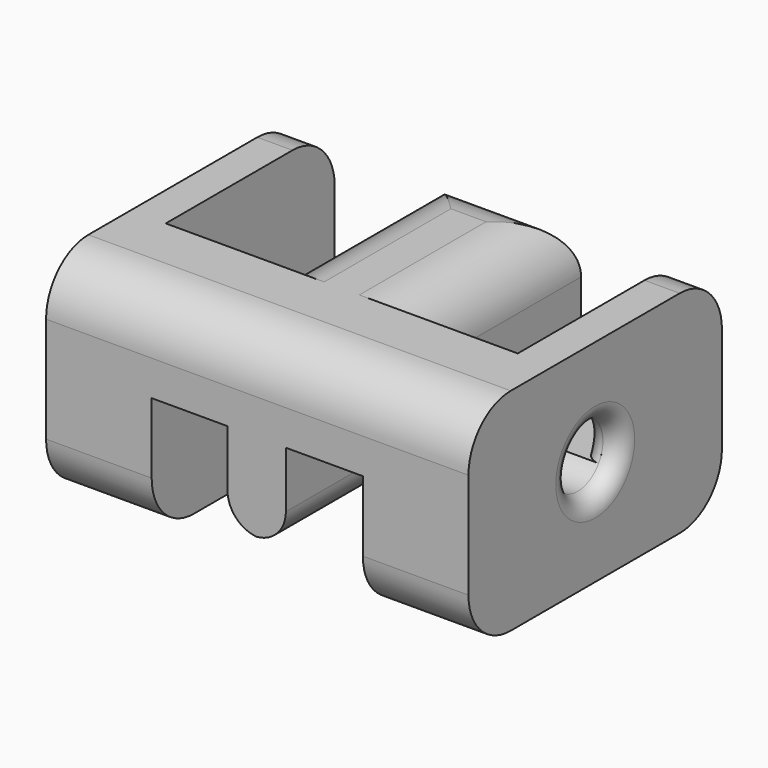
from build123d import *

# Parameters (mm, degrees)
F0_W         = 12
F0_H         = 9
F1_DEPTH     = 6
F2_W         = 3
F2_H         = 6
F3_DEPTH     = 3.5
F4_W         = 6
F4_H         = 6.5
F5_DEPTH     = 3.5
F6_R         = 0.9
F7_DEPTH     = 3
F8_R         = 0.9
F9_DEPTH     = 3.001
F10_R        = 1.5
F11_W        = 1.6597382491
F11_H        = 6.5
F12_DEPTH    = 2.5
F13_T1_DEPTH = 8.75
F14_R        = 0.49999


# Not quite as in the source:
# - a fillet or chamfer that OpenCascade refuses, or shapes differently, is made with other operations: its cross-section is extruded or revolved along the edge and cut away or added
# - a fillet or chamfer is up to 0.001 mm smaller than in the source, because OpenCascade refuses the exact size


with BuildPart() as f1:
    # F0 (on Top) → F1 (new body)
    with BuildSketch(Plane.XY):
        Rectangle(F0_W, F0_H)
    extrude(amount=F1_DEPTH)

    # F2 (on face) → F3 (cut)
    with BuildSketch(Plane.XY.offset(6)):
        with Locations((3.5, 1.5)):
            Rectangle(F2_W, F2_H)
        with Locations((-3.5, 1.5)):
            Rectangle(F2_W, F2_H)
    extrude(amount=-F3_DEPTH, mode=Mode.SUBTRACT)

    # F4 (on face) → F5 (cut)
    with BuildSketch(Plane(origin=(0, 0, 0), x_dir=(1, 0, 0), z_dir=(0, 0, -1))):
        with Locations((0, 1.25)):
            Rectangle(F4_W, F4_H)
    extrude(amount=-F5_DEPTH, mode=Mode.SUBTRACT)

    # F6 (on face) → F7 (cut)
    with BuildSketch(Plane.YZ.offset(6)):
        with Locations((0, 3)):
            Circle(F6_R)
    extrude(amount=-F7_DEPTH, mode=Mode.SUBTRACT)

    # F8 (on face) → F9 (cut, through all)
    with BuildSketch(Plane(origin=(-6, 0, 0), x_dir=(0, -1, 0), z_dir=(-1, 0, 0))):
        with Locations((0, 3)):
            Circle(F8_R)
    extrude(amount=-F9_DEPTH, mode=Mode.SUBTRACT)

    # F10
    f10_edges = [f1.edges().sort_by_distance(p)[0] for p in [
        (2, 1.5, 6),
        (-2, 1.5, 6),
        (0, -4.5, 6),
        (-4.5, -4.5, 0),
        (4.5, -4.5, 0),
        (0, 4.5, 0),
        (-5.5, 4.5, 6),
        (5.5, 4.5, 6),
        (0, 4.5, 6),
    ]]
    fillet(f10_edges, radius=F10_R)

    # F11 (on face) → F12 (join)
    with BuildSketch(Plane(origin=(0, 0, 3.5), x_dir=(1, 0, 0), z_dir=(0, 0, -1))):
        with Locations((-0.017724873, 1.25)):
            Rectangle(F11_W, F11_H)
    extrude(amount=F12_DEPTH)

    # F13: fillet of radius 0.9 on 2 edges, made by hand

    # F13_s2 → F13_t1 (cut)
    with BuildSketch(Plane.XZ.offset(-2)):
        with BuildLine():
            ThreePointArc((-0.0878557485, 1), (0.5485403546, 1.2636038969), (0.8121442515, 1.9))
            Line((0.8121442515, 1.9), (0.8121442515, 1))
            Line((0.8121442515, 1), (-0.0878557485, 1))
        make_face()
        with BuildLine():
            ThreePointArc((-0.8475939976, 1.9), (-0.5839901007, 1.2636038969), (0.0524060024, 1))
            Line((0.0524060024, 1), (-0.8475939976, 1))
            Line((-0.8475939976, 1), (-0.8475939976, 1.9))
        make_face()
    extrude(amount=F13_T1_DEPTH, mode=Mode.SUBTRACT)

    # F14 (radius 0.5 in the source; OpenCascade refuses exactly that, so slightly less here)
    f14_edges = [f1.edges().sort_by_distance(p)[0] for p in [
        (6, -0.9, 3),
        (-6, 0.9, 3),
        (-3, 0, 2.1),
        (5, 0.861249, 2.738751),
        (5, -0.261249, 3.861249),
        (3, 0, 2.1),
        (-5, -0.861249, 2.738751),
        (-5, 0.261249, 3.861249),
    ]]
    fillet(f14_edges, radius=F14_R)


solid = f1.part
